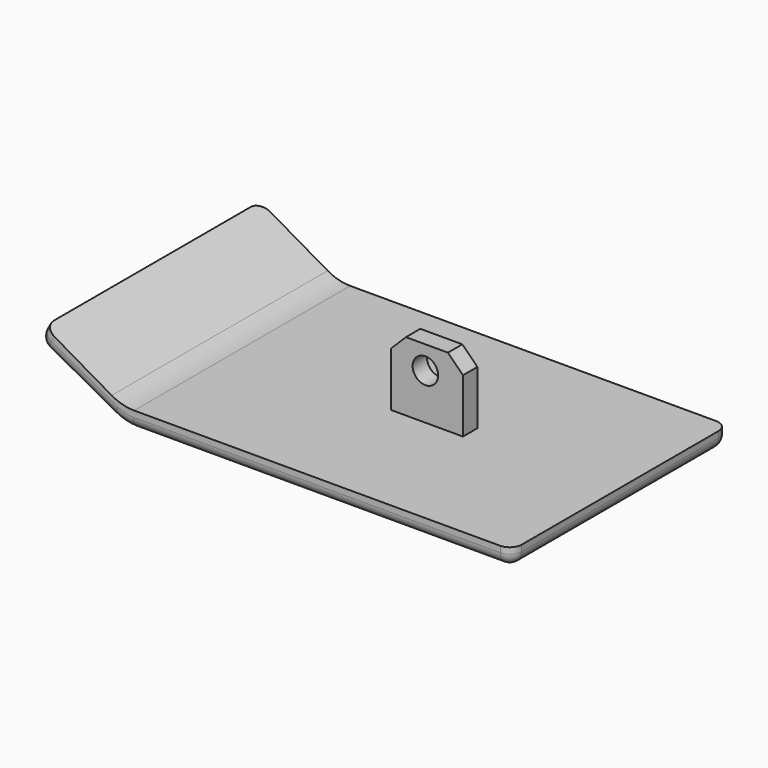
from build123d import *

# Parameters (mm, degrees)
F0_W         = 130
F0_H         = 6
F1_DEPTH     = 45
F2_R         = 15
F3_T1_DEPTH  = 39.0421058601
F3_T3_DEPTH  = 136.1787524098
F3_T6_ANGLE  = 28.601504949
F3_T8_ANGLE  = 28.601504949
F4_W         = 24
F4_H         = 6
F5_DEPTH     = 23
F6_SIZE      = 5
F7_R         = 4.25
F8_DEPTH     = 12.5
F9_T1_DEPTH  = 82.1112221979
F9_T3_DEPTH  = 12.0580253625
F9_T5_DEPTH  = 12.0580253625
F9_T8_ANGLE  = 88.3796937107
F9_T10_ANGLE = 88.3796937106
F9_T12_ANGLE = 88.3796937108
F9_T14_ANGLE = 88.3796937106
F10_R        = 1.65
F11_DEPTH    = 10
F12_DEPTH    = 10
F13_SIZE     = 1.7


# Not quite as in the source:
# - a fillet or chamfer that OpenCascade refuses, or shapes differently, is made with other operations: its cross-section is extruded or revolved along the edge and cut away or added


with BuildPart() as f1:
    # F0 (on Front) → F1 (new body, symmetric)
    with BuildSketch(Plane.XZ):
        Polygon((-28.8530516285, 15.7321775901), (0, 0), (0, 6), (-25.9807621135, 21), align=None)
        with Locations((65, 3)):
            Rectangle(F0_W, F0_H)
    extrude(amount=F1_DEPTH, both=True)

    # F2
    f2_edges = [f1.edges().sort_by_distance(p)[0] for p in [
        (0, 0, 6),
        (0, 0, 0),
    ]]
    fillet(f2_edges, radius=F2_R)

    # F3: fillet of radius 4 on 6 edges, made by hand

    # F3_s2 → F3_t1 (cut)
    with BuildSketch(Plane(origin=(-37.6348752969, 0, 20.5204825256), x_dir=(0, 1, 0), z_dir=(0.8779704017, 0, -0.4787149192))):
        with BuildLine():
            ThreePointArc((-45.0004, 4.0009656854), (-43.8284271247, 1.1715728753), (-40.9990343146, -0.0004))
            Line((-40.9990343146, -0.0004), (-40.9990343146, -0.4005365685))
            ThreePointArc((-40.9990343146, -0.4005365685), (-42.9995171573, -0.4001365685), (-45, -0.4001365685))
            Line((-45, -0.4001365685), (-45.4001365685, 0))
            ThreePointArc((-45.4001365685, 0), (-45.4001365685, 2.0004828427), (-45.4005365685, 4.0009656854))
            Line((-45.4005365685, 4.0009656854), (-45.0004, 4.0009656854))
        make_face()
        with BuildLine():
            ThreePointArc((45.0004, 4.0009656854), (43.8284271247, 1.1715728753), (40.9990343146, -0.0004))
            Line((40.9990343146, -0.0004), (40.9990343146, -0.4005365685))
            ThreePointArc((40.9990343146, -0.4005365685), (42.9995171573, -0.4001365685), (45, -0.4001365685))
            Line((45, -0.4001365685), (45.4001365685, 0))
            ThreePointArc((45.4001365685, 0), (45.4001365685, 2.0004828427), (45.4005365685, 4.0009656854))
            Line((45.4005365685, 4.0009656854), (45.0004, 4.0009656854))
        make_face()
    extrude(amount=F3_T1_DEPTH, mode=Mode.SUBTRACT)

    # F3_s4 → F3_t3 (cut)
    with BuildSketch(Plane.YZ.offset(3.8236618538)):
        with BuildLine():
            ThreePointArc((-45.0004, 4.0009656854), (-43.8284271247, 1.1715728753), (-40.9990343146, -0.0004))
            Line((-40.9990343146, -0.0004), (-40.9990343146, -0.4005365685))
            ThreePointArc((-40.9990343146, -0.4005365685), (-42.9995171573, -0.4001365685), (-45, -0.4001365685))
            Line((-45, -0.4001365685), (-45.4001365685, 0))
            ThreePointArc((-45.4001365685, 0), (-45.4001365685, 2.0004828427), (-45.4005365685, 4.0009656854))
            Line((-45.4005365685, 4.0009656854), (-45.0004, 4.0009656854))
        make_face()
        with BuildLine():
            ThreePointArc((45.0004, 4.0009656854), (43.8284271247, 1.1715728753), (40.9990343146, -0.0004))
            Line((40.9990343146, -0.0004), (40.9990343146, -0.4005365685))
            ThreePointArc((40.9990343146, -0.4005365685), (42.9995171573, -0.4001365685), (45, -0.4001365685))
            Line((45, -0.4001365685), (45.4001365685, 0))
            ThreePointArc((45.4001365685, 0), (45.4001365685, 2.0004828427), (45.4005365685, 4.0009656854))
            Line((45.4005365685, 4.0009656854), (45.0004, 4.0009656854))
        make_face()
    extrude(amount=F3_T3_DEPTH, mode=Mode.SUBTRACT)

    # F3_s5 → F3_t6 (revolve, cut)
    with BuildSketch(Plane.YZ.offset(3.8236618538)):
        with BuildLine():
            ThreePointArc((-45.0004, 4.0009656854), (-43.8284271247, 1.1715728753), (-40.9990343146, -0.0004))
            Line((-40.9990343146, -0.0004), (-40.9990343146, -0.4005365685))
            ThreePointArc((-40.9990343146, -0.4005365685), (-42.9995171573, -0.4001365685), (-45, -0.4001365685))
            Line((-45, -0.4001365685), (-45.4001365685, 0))
            ThreePointArc((-45.4001365685, 0), (-45.4001365685, 2.0004828427), (-45.4005365685, 4.0009656854))
            Line((-45.4005365685, 4.0009656854), (-45.0004, 4.0009656854))
        make_face()
    revolve(axis=Axis((3.8236618538, -45, 15), (0, 1, 0)), revolution_arc=F3_T6_ANGLE, mode=Mode.SUBTRACT)

    # F3_s7 → F3_t8 (revolve, cut)
    with BuildSketch(Plane.YZ.offset(3.8236618538)):
        with BuildLine():
            ThreePointArc((45.0004, 4.0009656854), (43.8284271247, 1.1715728753), (40.9990343146, -0.0004))
            Line((40.9990343146, -0.0004), (40.9990343146, -0.4005365685))
            ThreePointArc((40.9990343146, -0.4005365685), (42.9995171573, -0.4001365685), (45, -0.4001365685))
            Line((45, -0.4001365685), (45.4001365685, 0))
            ThreePointArc((45.4001365685, 0), (45.4001365685, 2.0004828427), (45.4005365685, 4.0009656854))
            Line((45.4005365685, 4.0009656854), (45.0004, 4.0009656854))
        make_face()
    revolve(axis=Axis((3.8236618538, 45, 15), (0, 1, 0)), revolution_arc=F3_T8_ANGLE, mode=Mode.SUBTRACT)

    # F9: fillet of radius 4 on 10 edges, made by hand

    # F9_s2 → F9_t1 (cut)
    with BuildSketch(Plane.XZ.offset(-41.0556110989)):
        with BuildLine():
            ThreePointArc((-26.938080852, 19.2450985259), (-27.2635959063, 16.1999344837), (-25.3405136646, 13.8165044373))
            Line((-25.3405136646, 13.8165044373), (-25.5320650096, 13.4651963735))
            ThreePointArc((-25.5320650096, 13.4651963735), (-27.2882382486, 14.423208544), (-29.0446029735, 15.3808695263))
            Line((-29.0446029735, 15.3808695263), (-29.2043596923, 15.9237289351))
            ThreePointArc((-29.2043596923, 15.9237289351), (-28.2466987099, 17.6800936601), (-27.2893889158, 19.4366498709))
            Line((-27.2893889158, 19.4366498709), (-26.938080852, 19.2450985259))
        make_face()
        with BuildLine():
            ThreePointArc((130.0004, 4.0009656854), (128.8284271247, 1.1715728753), (125.9990343146, -0.0004))
            Line((125.9990343146, -0.0004), (125.9990343146, -0.4005365685))
            ThreePointArc((125.9990343146, -0.4005365685), (127.9995171573, -0.4001365685), (130, -0.4001365685))
            Line((130, -0.4001365685), (130.4001365685, 0))
            ThreePointArc((130.4001365685, 0), (130.4001365685, 2.0004828427), (130.4005365685, 4.0009656854))
            Line((130.4005365685, 4.0009656854), (130.0004, 4.0009656854))
        make_face()
    extrude(amount=F9_T1_DEPTH, mode=Mode.SUBTRACT)

    # F9_s4 → F9_t3 (cut)
    with BuildSketch(Plane(origin=(7.6605944504, 0, 14.0496460784), x_dir=(0, 1, 0), z_dir=(-0.4787149192, 0, -0.8779704017))):
        with BuildLine():
            ThreePointArc((45.0004, -28.8623877649), (43.8284271247, -31.6917805751), (40.9990343146, -32.8637534503))
            Line((40.9990343146, -32.8637534503), (40.9990343146, -33.2638900189))
            ThreePointArc((40.9990343146, -33.2638900189), (42.9995171573, -33.2634900189), (45, -33.2634900189))
            Line((45, -33.2634900189), (45.4001365685, -32.8633534503))
            ThreePointArc((45.4001365685, -32.8633534503), (45.4001365685, -30.8628706076), (45.4005365685, -28.8623877649))
            Line((45.4005365685, -28.8623877649), (45.0004, -28.8623877649))
        make_face()
        with BuildLine():
            ThreePointArc((-40.9990343146, -32.8637534503), (-43.8284271247, -31.6917805751), (-45.0004, -28.8623877649))
            Line((-45.0004, -28.8623877649), (-45.4005365685, -28.8623877649))
            ThreePointArc((-45.4005365685, -28.8623877649), (-45.4001365685, -30.8628706076), (-45.4001365685, -32.8633534503))
            Line((-45.4001365685, -32.8633534503), (-45, -33.2634900189))
            ThreePointArc((-45, -33.2634900189), (-42.9995171573, -33.2634900189), (-40.9990343146, -33.2638900189))
            Line((-40.9990343146, -33.2638900189), (-40.9990343146, -32.8637534503))
        make_face()
    extrude(amount=F9_T3_DEPTH, mode=Mode.SUBTRACT)

    # F9_s6 → F9_t5 (cut)
    with BuildSketch(Plane.XY.offset(3.9443889011)):
        with BuildLine():
            ThreePointArc((125.9990343146, 45.0004), (128.8284271247, 43.8284271247), (130.0004, 40.9990343146))
            Line((130.0004, 40.9990343146), (130.4005365685, 40.9990343146))
            ThreePointArc((130.4005365685, 40.9990343146), (130.4001365685, 42.9995171573), (130.4001365685, 45))
            Line((130.4001365685, 45), (130, 45.4001365685))
            ThreePointArc((130, 45.4001365685), (127.9995171573, 45.4001365685), (125.9990343146, 45.4005365685))
            Line((125.9990343146, 45.4005365685), (125.9990343146, 45.0004))
        make_face()
        with BuildLine():
            ThreePointArc((125.9990343146, -45.0004), (128.8284271247, -43.8284271247), (130.0004, -40.9990343146))
            Line((130.0004, -40.9990343146), (130.4005365685, -40.9990343146))
            ThreePointArc((130.4005365685, -40.9990343146), (130.4001365685, -42.9995171573), (130.4001365685, -45))
            Line((130.4001365685, -45), (130, -45.4001365685))
            ThreePointArc((130, -45.4001365685), (127.9995171573, -45.4001365685), (125.9990343146, -45.4005365685))
            Line((125.9990343146, -45.4005365685), (125.9990343146, -45.0004))
        make_face()
    extrude(amount=F9_T5_DEPTH, mode=Mode.SUBTRACT)

    # F9_s7 → F9_t8 (revolve, cut)
    with BuildSketch(Plane(origin=(0.2778664319, -41.0474031895, 0.5096112384), x_dir=(-0.9999770884, -0.0067692483, 0), z_dir=(-0.0067687267, 0.9999000341, -0.0124139472))):
        with BuildLine():
            ThreePointArc((27.2151878021, 18.7365799005), (27.5408308098, 15.6914295387), (25.6178487183, 13.3079186891))
            Line((25.6178487183, 13.3079186891), (25.8094148247, 12.9566186743))
            ThreePointArc((25.8094148247, 12.9566186743), (27.5655478077, 13.914704636), (29.3218722914, 14.8724394175))
            Line((29.3218722914, 14.8724394175), (29.4816061998, 15.4153055387))
            ThreePointArc((29.4816061998, 15.4153055387), (28.5238714183, 17.1716300224), (27.5664878169, 18.9281460069))
            Line((27.5664878169, 18.9281460069), (27.2151878021, 18.7365799005))
        make_face()
    revolve(axis=Axis((-26.9377296637, -40.9990343144, 19.2449070401), (-0.8779704017, 0, 0.4787149192)), revolution_arc=F9_T8_ANGLE, mode=Mode.SUBTRACT)

    # F9_s9 → F9_t10 (revolve, cut)
    with BuildSketch(Plane(origin=(2.1924225676, 0.0647620721, 4.0209361465), x_dir=(-0.0295261677, 0.9995640077, 0), z_dir=(0.478667064, 0.0141393687, 0.8778826346))):
        with BuildLine():
            ThreePointArc((41.7769372077, 31.7914495116), (44.5749980004, 30.5465238532), (45.673230386, 27.6877007173))
            Line((45.673230386, 27.6877007173), (46.0732324846, 27.6773279365))
            ThreePointArc((46.0732324846, 27.6773279365), (46.1246913384, 29.6771488661), (46.1765500578, 31.6769594264))
            Line((46.1765500578, 31.6769594264), (45.7869207399, 32.0873343059))
            ThreePointArc((45.7869207399, 32.0873343059), (43.7871101796, 32.1391930252), (41.7873099885, 32.1914516102))
            Line((41.7873099885, 32.1914516102), (41.7769372077, 31.7914495116))
        make_face()
    revolve(axis=Axis((-26.9377296637, 40.9990343144, 19.2449070401), (-0.8779704017, 0, 0.4787149192)), revolution_arc=F9_T10_ANGLE, mode=Mode.SUBTRACT)

    # F9_s11 → F9_t12 (revolve, cut)
    with BuildSketch(Plane(origin=(0, -41.0474031895, 0.5804423901), x_dir=(1, 0, 0), z_dir=(0, 0.9999000341, -0.0141393686))):
        with BuildLine():
            ThreePointArc((130.0004, -3.420465265), (128.8284271247, -0.5910724549), (125.9990343146, 0.5809004204))
            Line((125.9990343146, 0.5809004204), (125.9990343146, 0.9810369889))
            ThreePointArc((125.9990343146, 0.9810369889), (127.9995171573, 0.9806369889), (130, 0.9806369889))
            Line((130, 0.9806369889), (130.4001365685, 0.5805004204))
            ThreePointArc((130.4001365685, 0.5805004204), (130.4001365685, -1.4199824223), (130.4005365685, -3.420465265))
            Line((130.4005365685, -3.420465265), (130.0004, -3.420465265))
        make_face()
    revolve(axis=Axis((130, -40.9990343144, 4.0009656856), (-1, 0, 0)), revolution_arc=F9_T12_ANGLE, mode=Mode.SUBTRACT)

    # F9_s13 → F9_t14 (revolve, cut)
    with BuildSketch(Plane(origin=(0, 0.0647620721, 4.5798083157), x_dir=(1, 0, 0), z_dir=(0, 0.0141393687, 0.9999000341))):
        with BuildLine():
            ThreePointArc((130.0004, 40.9387646817), (128.8284271247, 43.7681574918), (125.9990343146, 44.9401303671))
            Line((125.9990343146, 44.9401303671), (125.9990343146, 45.3402669356))
            ThreePointArc((125.9990343146, 45.3402669356), (127.9995171573, 45.3398669356), (130, 45.3398669356))
            Line((130, 45.3398669356), (130.4001365685, 44.9397303671))
            ThreePointArc((130.4001365685, 44.9397303671), (130.4001365685, 42.9392475244), (130.4005365685, 40.9387646817))
            Line((130.4005365685, 40.9387646817), (130.0004, 40.9387646817))
        make_face()
    revolve(axis=Axis((130, 40.9990343144, 4.0009656856), (-1, 0, 0)), revolution_arc=F9_T14_ANGLE, mode=Mode.SUBTRACT)

    # F10 (on face) → F12 (cut)
    with BuildSketch(Plane.XY.offset(6)):
        with Locations((75, 0)):
            Circle(F10_R)
        with Locations((61, 0)):
            Circle(F10_R)
        with Locations((68, 0)):
            Circle(F10_R)
    extrude(amount=-F12_DEPTH, mode=Mode.SUBTRACT)

    # F13
    f13_edges = [f1.edges().sort_by_distance(p)[0] for p in [
        (59.35, 0, 0),
        (66.35, 0, 0),
        (73.35, 0, 0),
        (3.823662, 0, 0),
        (64.939636, 41.055611, 0),
        (64.939636, -41.055611, 0),
        (126.055611, 0, 0),
    ]]
    chamfer(f13_edges, length=F13_SIZE)


with BuildPart() as f5:
    # F4 (on face) → F5 (new body)
    with BuildSketch(Plane.XY.offset(6)):
        with Locations((68, 0)):
            Rectangle(F4_W, F4_H)
    extrude(amount=F5_DEPTH)

    # F6
    f6_edges = [f5.edges().sort_by_distance(p)[0] for p in [
        (80, 0, 29),
        (56, 0, 29),
    ]]
    chamfer(f6_edges, length=F6_SIZE)

    # F7 (on face) → F8 (cut, symmetric)
    with BuildSketch(Plane(origin=(0, 3, 0), x_dir=(-1, 0, 0), z_dir=(0, 1, 0))):
        with Locations((-67.4792453647, 21.25)):
            Circle(F7_R)
    extrude(amount=F8_DEPTH, both=True, mode=Mode.SUBTRACT)

    # F10 (on face) → F11 (cut)
    with BuildSketch(Plane.XY.offset(6)):
        with Locations((75, 0)):
            Circle(F10_R)
        with Locations((68, 0)):
            Circle(F10_R)
        with Locations((61, 0)):
            Circle(F10_R)
    extrude(amount=F11_DEPTH, mode=Mode.SUBTRACT)


solid = Compound([f1.part, f5.part])
